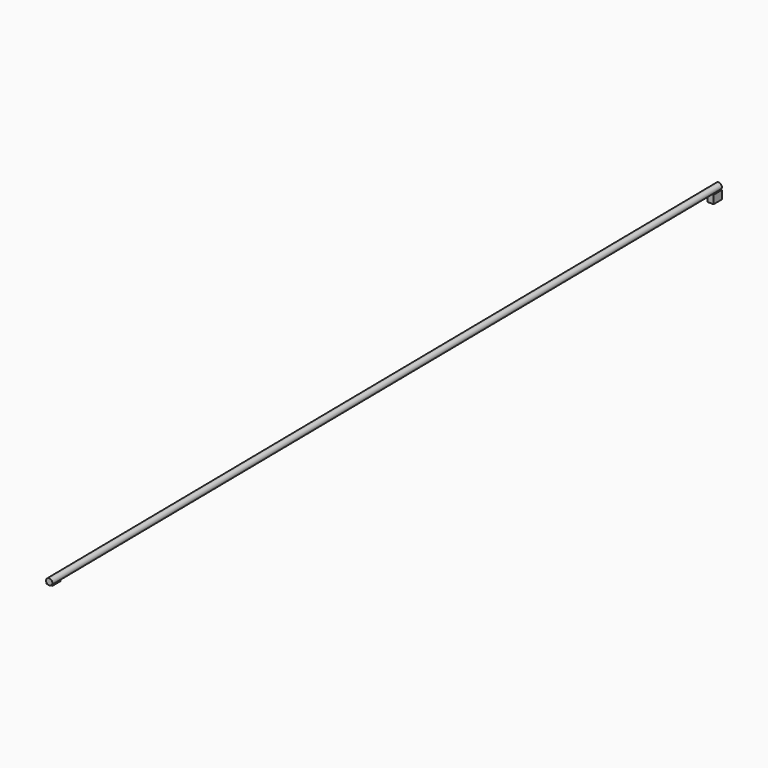
from build123d import *

# Parameters (mm, degrees)
F1_DEPTH = 60
F2_R     = 30
F3_DEPTH = 8000


with BuildPart() as f1:
    # F0 (on Right) → F1 (new body)
    with BuildSketch(Plane.YZ):
        Polygon((100, 1), (0, 0), (100, 0), align=None)
    extrude(amount=F1_DEPTH)


with BuildPart() as f1b:
    # F0 (on Right) → F1, piece 2 (new body)
    with BuildSketch(Plane.YZ):
        Polygon((7999.200079992, 79.9920007999), (7900, 79), (7900, 0), (8000, 0), align=None)
    extrude(amount=F1_DEPTH)

    # F2 (on face) → F3 (join)
    with BuildSketch(Plane(origin=(0, 7999.200079992, 79.9920007999), x_dir=(-1, 0, 0), z_dir=(0, 0.9999500037, 0.0099995))):
        with Locations((-30, 25.0039997)):
            Circle(F2_R)
    extrude(amount=-F3_DEPTH)


solid = Compound([f1.part, f1b.part])
